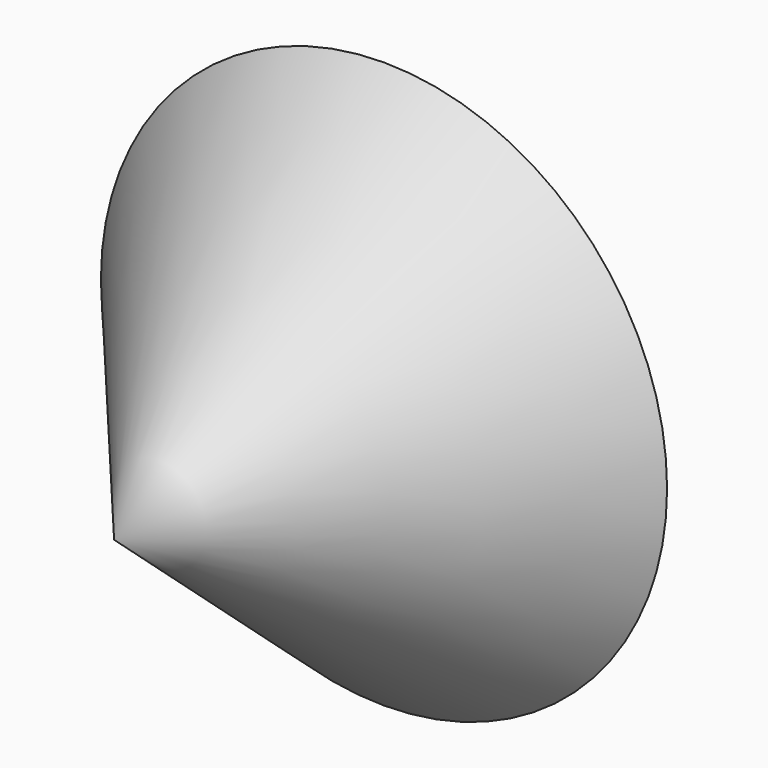
from build123d import *

# Parameters (mm, degrees)
F0_R = 38.2977843127


# Not quite as in the source:
# - an extrude whose draft closes it to a point is written as a loft to that point


with BuildPart() as f1:
    # F0 (on Front) → F1 section 0
    with BuildSketch(Plane.XZ, mode=Mode.PRIVATE) as f1_s0:
        Circle(F0_R)
    loft([f1_s0.sketch, Vertex(0, -45.6415220431, 0)], ruled=True)


solid = f1.part
